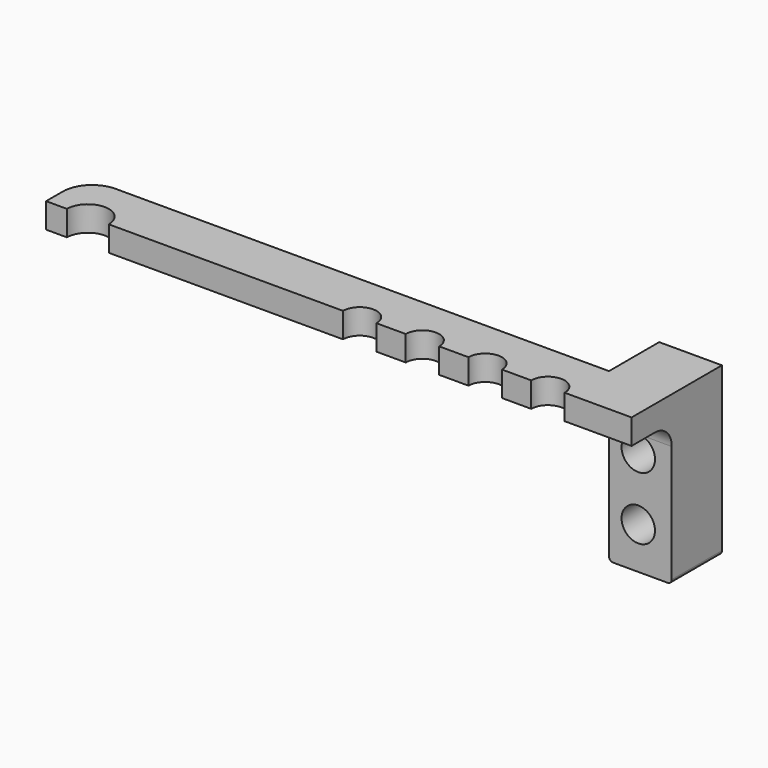
from build123d import *

# Parameters (mm, degrees)
F1_DEPTH = 6
F2_R     = 7
F3_W     = 15
F3_H     = 34
F3_H_2   = 6
F4_DEPTH = 15
F5_R     = 4
F6_DEPTH = 25
F7_R     = 4.99999
F8_R     = 1


# Not quite as in the source:
# - a fillet or chamfer is up to 0.001 mm smaller than in the source, because OpenCascade refuses the exact size


with BuildPart() as f1:
    # F0 (on Top) → F1 (new body)
    with BuildSketch(Plane.XY):
        with BuildLine():
            ThreePointArc((-70, 0), (-65, 5), (-60, 0))
            Line((-60, 0), (-4, 0))
            ThreePointArc((-4, 0), (0, 4), (4, 0))
            Line((4, 0), (11, 0))
            ThreePointArc((11, 0), (15, 4), (19, 0))
            Line((19, 0), (26, 0))
            ThreePointArc((26, 0), (30, 4), (34, 0))
            Line((34, 0), (41, 0))
            ThreePointArc((41, 0), (45, 4), (49, 0))
            Line((49, 0), (65, 0))
            Line((65, 0), (65, 12))
            Line((65, 12), (-75, 12))
            Line((-75, 12), (-75, 0))
            Line((-75, 0), (-70, 0))
        make_face()
    extrude(amount=F1_DEPTH)

    # F2
    f2_edges = [f1.edges().sort_by_distance(p)[0] for p in [
        (-75, 12, 3),
    ]]
    fillet(f2_edges, radius=F2_R)

    # F3 (on face) → F4 (join)
    with BuildSketch(Plane(origin=(0, 12, 0), x_dir=(-1, 0, 0), z_dir=(0, 1, 0))):
        with Locations((-57.5, -17)):
            Rectangle(F3_W, F3_H)
        with Locations((-57.5, 3)):
            Rectangle(F3_W, F3_H_2)
    extrude(amount=F4_DEPTH)

    # F5 (on face) → F6 (cut)
    with BuildSketch(Plane.XZ.offset(-12)):
        with Locations((57, -9)):
            Circle(F5_R)
        with Locations((57, -24)):
            Circle(F5_R)
    extrude(amount=-F6_DEPTH, mode=Mode.SUBTRACT)

    # F7 (radius 5 in the source; OpenCascade refuses exactly that, so slightly less here)
    f7_edges = [f1.edges().sort_by_distance(p)[0] for p in [
        (57.5, 12, 0),
    ]]
    fillet(f7_edges, radius=F7_R)

    # F8
    f8_edges = [f1.edges().sort_by_distance(p)[0] for p in [
        (65, 19.5, -34),
        (50, 19.5, -34),
    ]]
    fillet(f8_edges, radius=F8_R)


solid = f1.part
